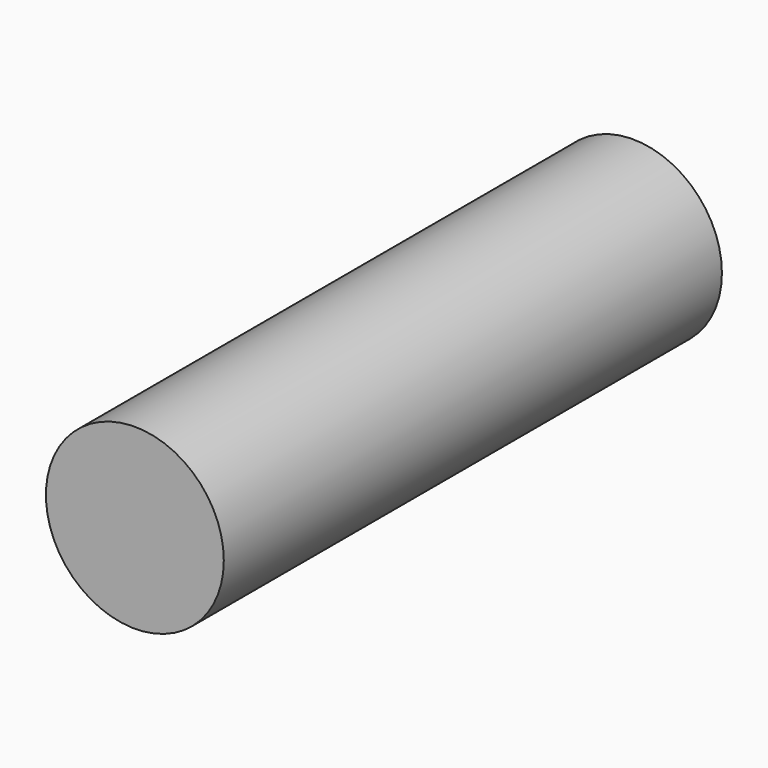
from build123d import *

# Parameters (mm, degrees)
F0_R     = 3.175
F1_DEPTH = 22.225


# Not quite as in the source:
# - an extrude whose draft closes it to a point is written as a loft to that point


with BuildPart() as f1:
    # F0 (on Front) → F1 (new body)
    with BuildSketch(Plane.XZ):
        Circle(F0_R)
    extrude(amount=F1_DEPTH)

    # F0 (on Front) → F2 section 0
    with BuildSketch(Plane.XZ, mode=Mode.PRIVATE) as f2_s0:
        Circle(F0_R)
    loft([f2_s0.sketch, Vertex(0, 1.5829966056, 0)], ruled=True)


solid = f1.part
